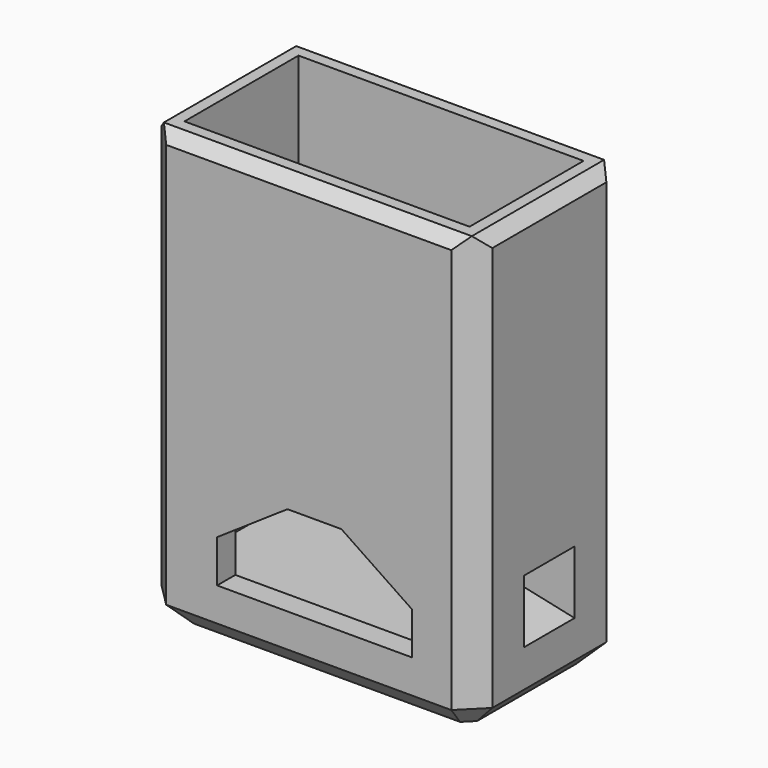
from build123d import *

# Parameters (mm, degrees)
F0_W      = 29
F0_H      = 16.5
F1_DEPTH  = 38.5
F2_T      = -2
F3_DEPTH  = 2.5
F4_SIZE   = 2
F5_SIZE   = 2
F6_SIZE   = 0.99999
F8_DEPTH  = 16.501
F9_W      = 7.54
F9_H      = 7.25
F9_R      = 1.1
F10_DEPTH = 6.35
F13_W     = 5.538
F13_H     = 4.583
F11_W     = 5.533
F11_H     = 5.533


# Not quite as in the source:
# - a fillet or chamfer is up to 0.001 mm smaller than in the source, because OpenCascade refuses the exact size


with BuildPart() as f1:
    # F0 (on Top) → F1 (new body)
    with BuildSketch(Plane.XY):
        with Locations((14.5, 8.25)):
            Rectangle(F0_W, F0_H)
    extrude(amount=F1_DEPTH)

    # F2
    f2_openings = [f1.faces().sort_by_distance(p)[0] for p in [
        (14.5, 8.25, 38.5),
    ]]
    offset(amount=F2_T, openings=f2_openings)

    # F3 (add): a face of the model
    f3_faces = [f1.faces().sort_by_distance(p)[0] for p in [
        (14.5, 8.25, 2),
    ]]
    extrude(f3_faces, amount=F3_DEPTH)

    # F4
    f4_edges = [f1.edges().sort_by_distance(p)[0] for p in [
        (29, 0, 19.25),
        (29, 16.5, 19.25),
        (0, 0, 19.25),
        (0, 16.5, 19.25),
    ]]
    chamfer(f4_edges, length=F4_SIZE)

    # F5
    f5_edges = [f1.edges().sort_by_distance(p)[0] for p in [
        (0, 8.25, 0),
        (1, 15.5, 0),
        (1, 1, 0),
        (14.5, 16.5, 0),
        (14.5, 0, 0),
        (28, 15.5, 0),
        (28, 1, 0),
        (29, 8.25, 0),
    ]]
    chamfer(f5_edges, length=F5_SIZE)

    # F6 (size 1 in the source; OpenCascade refuses exactly that, so slightly less here)
    f6_edges = [f1.edges().sort_by_distance(p)[0] for p in [
        (14.5, 16.5, 38.5),
        (0, 8.25, 38.5),
        (14.5, 0, 38.5),
        (29, 8.25, 38.5),
    ]]
    chamfer(f6_edges, length=F6_SIZE)

    # F7 (on face) → F8 (cut, through all)
    with BuildSketch(Plane.XZ):
        Polygon((12.635, 12.834), (6.464, 8.667), (6.464, 4.94), (23.536, 4.94), (23.536, 8.667), (17.365, 12.834), align=None)
    extrude(amount=-F8_DEPTH, mode=Mode.SUBTRACT)

    # F9 (on face) → F10 (join)
    with BuildSketch(Plane.YZ.offset(29)):
        with Locations((8.25, 7.875)):
            Rectangle(F9_W, F9_H)
        with Locations((8.25, 9)):
            Circle(F9_R, mode=Mode.SUBTRACT)
    extrude(amount=-F10_DEPTH)

    # F13 (on offset) → F14 section 0
    with BuildSketch(Plane.YZ.offset(24.55)):
        with Locations((8.258, 8.5135)):
            Rectangle(F13_W, F13_H)
    # F11 (on face) → F14 section 1
    with BuildSketch(Plane.YZ.offset(29)):
        with Locations((8.2475, 8.0385)):
            Rectangle(F11_W, F11_H)
    loft(mode=Mode.SUBTRACT)


solid = f1.part
